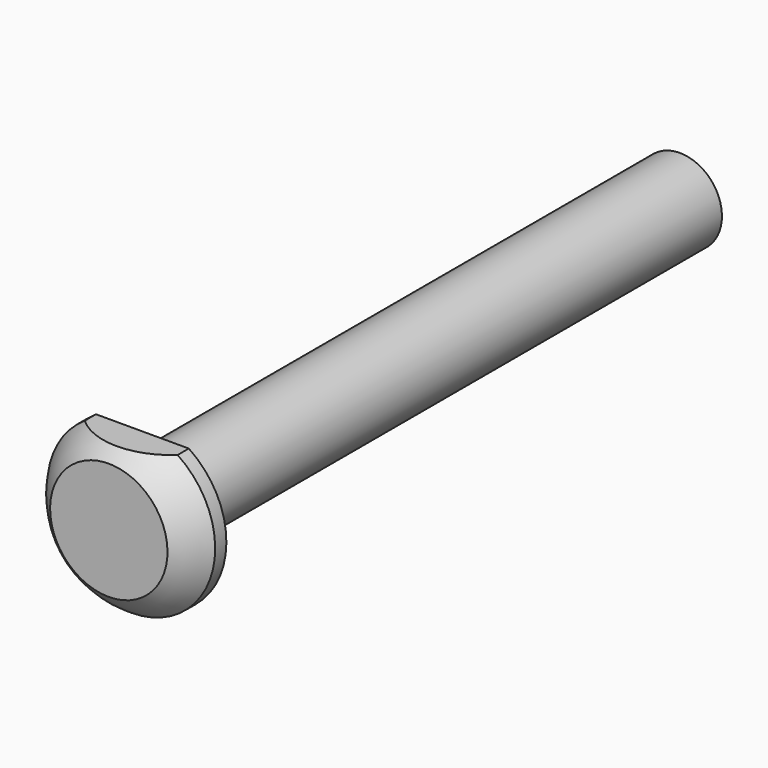
from build123d import *

# Parameters (mm, degrees)
F3_DEPTH = 4.7635


with BuildPart() as f1:
    # F0 (on Right) → F1 (revolve)
    with BuildSketch(Plane.YZ):
        Polygon((27.2266382913, 0), (0, 0), (-44.8370490589, 0), (-48.9733617087, 0), (-48.9733617087, -4.7625), (27.2266382913, -4.7625), align=None)
        with BuildLine():
            Line((-48.9733617087, -4.7625), (-48.9733617087, 0))
            Line((-48.9733617087, 0), (-53.7358617087, 0))
            Line((-53.7358617087, 0), (-53.7358617087, -6.655733594))
            ThreePointArc((-53.7358617087, -6.655733594), (-52.2877849347, -8.2446462119), (-50.5608617087, -9.525))
            Line((-50.5608617087, -9.525), (-48.9733617087, -9.525))
            Line((-48.9733617087, -9.525), (-48.9733617087, -4.7625))
        make_face()
    revolve(axis=Axis((0, -10.8733617087, 0), (0, -1, 0)))

    # F2 (on face) → F3 (cut, through all)
    with BuildSketch(Plane(origin=(0, -48.9733617087, 0), x_dir=(-1, 0, 0), z_dir=(0, 1, 0))):
        with BuildLine():
            Line((-5.2651418547, 7.9375), (0, 7.9375))
            Line((0, 7.9375), (5.2651418547, 7.9375))
            ThreePointArc((5.2651418547, 7.9375), (0, 9.525), (-5.2651418547, 7.9375))
        make_face()
    extrude(amount=-F3_DEPTH, mode=Mode.SUBTRACT)


solid = f1.part
